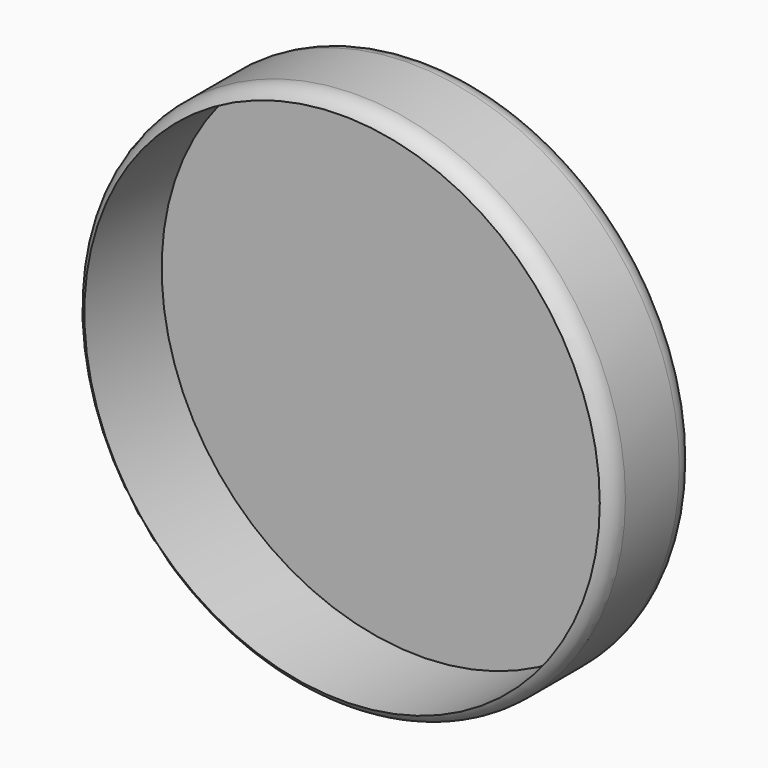
from build123d import *

# Parameters (mm, degrees)
F0_R     = 63.5
F1_DEPTH = 25.4
F2_T     = -2.54


# Not quite as in the source:
# - a fillet or chamfer that OpenCascade refuses, or shapes differently, is made with other operations: its cross-section is extruded or revolved along the edge and cut away or added


with BuildPart() as f1:
    # F0 (on Front) → F1 (new body)
    with BuildSketch(Plane.XZ):
        Circle(F0_R)
    extrude(amount=F1_DEPTH)

    # F2
    f2_openings = [f1.faces().sort_by_distance(p)[0] for p in [
        (0, -25.4, 0),
    ]]
    offset(amount=F2_T, openings=f2_openings)

    # F3: fillet of radius 5.08 on 3 edges, made by hand

    # F3_s1 → F3_t2 (revolve, cut)
    with BuildSketch(Plane.XY):
        with BuildLine():
            ThreePointArc((63.5, -5.08), (62.0121024484, -1.4878975516), (58.42, 0))
            Line((58.42, 0), (63.5, 0))
            Line((63.5, 0), (63.5, -5.08))
        make_face()
    revolve(axis=Axis((0, 0, 0), (0, -1, 0)), mode=Mode.SUBTRACT)

    # F3_s3 → F3_t4 (revolve, cut)
    with BuildSketch(Plane.XY):
        with BuildLine():
            ThreePointArc((63.5, -21.0005909488), (62.8194090512, -23.5405909488), (60.96, -25.4))
            Line((60.96, -25.4), (63.5, -25.4))
            Line((63.5, -25.4), (63.5, -21.0005909488))
        make_face()
    revolve(axis=Axis((0, -25.4, 0), (0, -1, 0)), mode=Mode.SUBTRACT)


solid = f1.part
